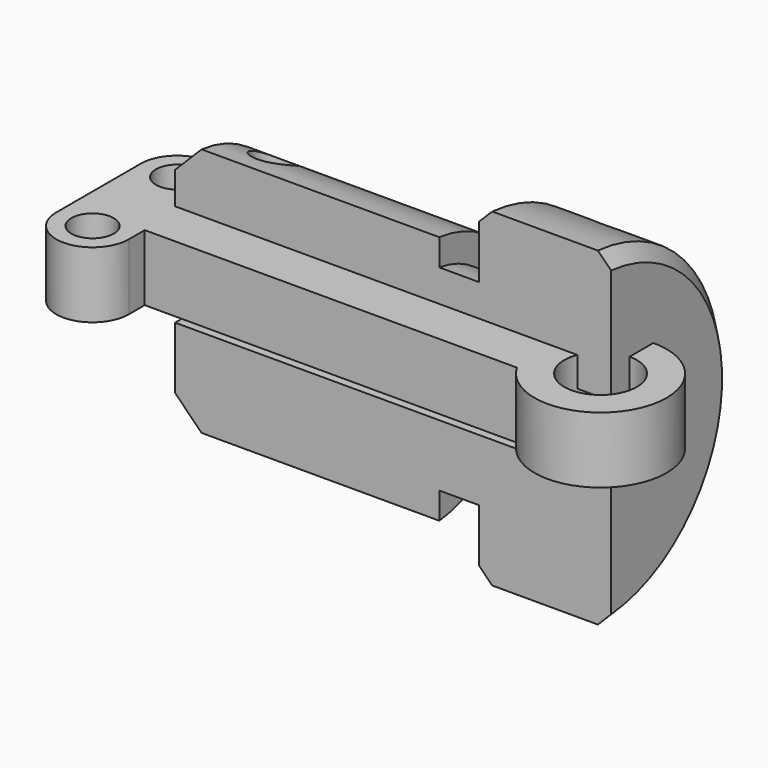
from build123d import *

# Parameters (mm, degrees)
F1_ANGLE    = 180
F3_DEPTH    = 33.001
F4_W        = 6
F4_H        = 5.5
F5_DEPTH    = 10
F6_W        = 1.5
F6_H        = 5.5
F7_DEPTH    = 23.001
F8_T2_ANGLE = 230.0428222626
F9_R        = 1.5
F10_DEPTH   = 12.5
F11_R       = 1.6
F11_R_2     = 2.75
F12_DEPTH   = 5
F13_SIZE    = 1
F15_R       = 2.75
F16_DEPTH   = 5.3450514045


# Not quite as in the source:
# - a fillet or chamfer that OpenCascade refuses, or shapes differently, is made with other operations: its cross-section is extruded or revolved along the edge and cut away or added


with BuildPart() as f1:
    # F0 (on Front) → F1 (revolve)
    with BuildSketch(Plane.XZ):
        Polygon((-33, 0), (0, 0), (0, 12.5), (-10, 12.5), (-10, 7.5), (-13, 7.5), (-13, 9.5), (-33, 9.5), align=None)
    revolve(axis=Axis((-16.5, 0, 0), (-1, 0, 0)), revolution_arc=F1_ANGLE)

    # F2 (on face) → F3 (cut, through all)
    with BuildSketch(Plane.YZ):
        with BuildLine():
            ThreePointArc((1, 12.4599357944), (0.5004011242, 12.4899799325), (0, 12.5))
            Line((0, 12.5), (0, -12.5))
            ThreePointArc((0, -12.5), (0.5004011242, -12.4899799325), (1, -12.4599357944))
            Line((1, -12.4599357944), (1, 12.4599357944))
        make_face()
        with BuildLine():
            ThreePointArc((1, -12.4599357944), (0.5004011242, -12.4899799325), (0, -12.5))
            Line((0, -12.5), (0, -17.5))
            Line((0, -17.5), (1, -17.5))
            Line((1, -17.5), (1, -12.4599357944))
        make_face()
    extrude(amount=-F3_DEPTH, mode=Mode.SUBTRACT)

    # F4 (on face) → F5 (cut)
    with BuildSketch(Plane(origin=(-33, 0, 0), x_dir=(0, -1, 0), z_dir=(-1, 0, 0))):
        with Locations((-4, 0)):
            Rectangle(F4_W, F4_H)
    extrude(amount=-F5_DEPTH, mode=Mode.SUBTRACT)

    # F6 (on face) → F7 (cut, through all)
    with BuildSketch(Plane(origin=(-23, 0, 0), x_dir=(0, -1, 0), z_dir=(-1, 0, 0))):
        with Locations((-1.75, 0)):
            Rectangle(F6_W, F6_H)
    extrude(amount=-F7_DEPTH, mode=Mode.SUBTRACT)

    # F8: chamfer of 2 on 1 edges, made by hand

    # F8_s1 → F8_t2 (revolve, cut)
    with BuildSketch(Plane(origin=(0, 0, 0), x_dir=(1, 0, 0), z_dir=(0, -0.9061497935, -0.4229569147))):
        Polygon((-31, 9.5), (-33, 7.5), (-33, 9.5), align=None)
    revolve(axis=Axis((-33, 0, 0), (-1, 0, 0)), revolution_arc=F8_T2_ANGLE, mode=Mode.SUBTRACT)

    # F9 (on Top) → F10 (cut, symmetric)
    with BuildSketch(Plane.XY):
        with Locations((-28, 4)):
            Circle(F9_R)
    extrude(amount=F10_DEPTH, both=True, mode=Mode.SUBTRACT)

    # F13
    f13_edges = [f1.edges().sort_by_distance(p)[0] for p in [
        (-10, 12.5, 0),
        (0, 12.5, 0),
    ]]
    chamfer(f13_edges, length=F13_SIZE)

    # F15 (on offset) → F16 (cut, through all)
    with BuildSketch(Plane.XZ.offset(-6)):
        with Locations((-5, -8)):
            Circle(F15_R)
        with Locations((-5, 8)):
            Circle(F15_R)
    extrude(amount=-F16_DEPTH, mode=Mode.SUBTRACT)


with BuildPart() as f12:
    # F11 (on Top) → F12 (new body)
    with BuildSketch(Plane.XY):
        with BuildLine():
            Line((-32.5, -2.5), (-4.3301270189, -2.5))
            ThreePointArc((-4.3301270189, -2.5), (5, 0), (-4.3301270189, 2.5))
            Line((-4.3301270189, 2.5), (-32.5, 2.5))
            Line((-32.5, 2.5), (-32.5, 4))
            ThreePointArc((-32.5, 4), (-35.25, 6.75), (-38, 4))
            Line((-38, 4), (-38, -4))
            ThreePointArc((-38, -4), (-35.25, -6.75), (-32.5, -4))
            Line((-32.5, -4), (-32.5, -2.5))
        make_face()
        with Locations((-35.25, -4)):
            Circle(F11_R, mode=Mode.SUBTRACT)
        with Locations((-35.25, 4)):
            Circle(F11_R, mode=Mode.SUBTRACT)
        Circle(F11_R_2, mode=Mode.SUBTRACT)
    extrude(amount=F12_DEPTH)


solid = Compound([f1.part, f12.part])
